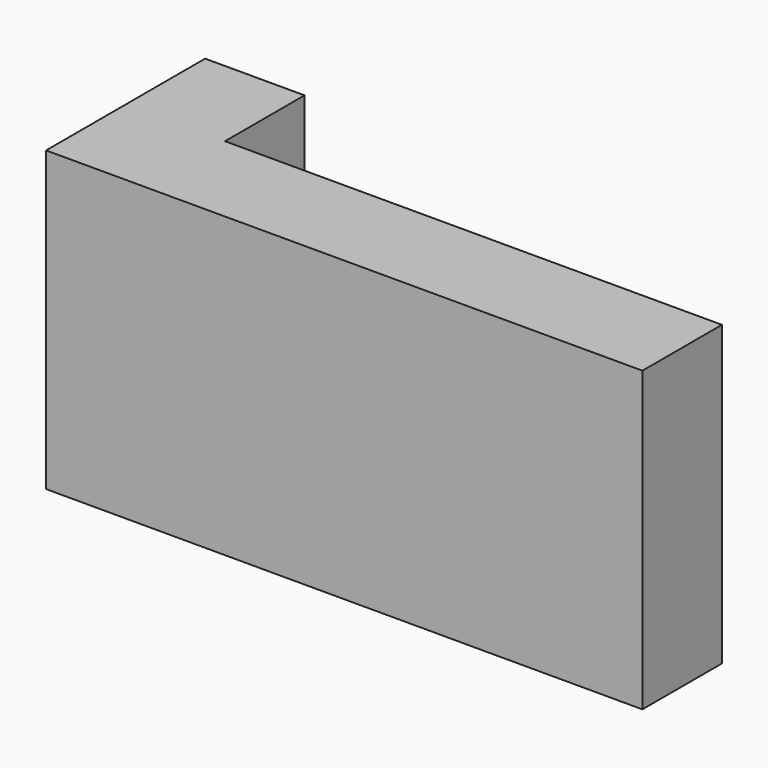
from build123d import *

# Parameters (mm, degrees)
F1_DEPTH = 50.8
F2_DEPTH = 25.4
F3_DEPTH = 25.4


with BuildPart() as f1:
    # F0 (on Top) → F1 (new body)
    with BuildSketch(Plane.XY):
        Polygon((-37.0331916732, 55.9852184538), (-62.4331916732, 55.9852184538), (-62.4331916732, 5.1852184538), (89.9668083268, 5.1852184538), (89.9668083268, 30.5852184538), (-37.0331916732, 30.5852184538), (-37.0331916732, 55.3826626255), align=None)
    extrude(amount=-F1_DEPTH)

    # F0 (on Top) → F3 (join)
    with BuildSketch(Plane.XY):
        Polygon((-37.0331916732, 55.9852184538), (-62.4331916732, 55.9852184538), (-62.4331916732, 5.1852184538), (89.9668083268, 5.1852184538), (89.9668083268, 30.5852184538), (-37.0331916732, 30.5852184538), (-37.0331916732, 55.3826626255), align=None)
    extrude(amount=F3_DEPTH)


with BuildPart() as f2:
    # F0 (on Top) → F2 (new body)
    with BuildSketch(Plane.XY):
        Polygon((89.9668083268, 30.5852184538), (-37.0331916732, 55.3826626255), (-37.0331916732, 30.5852184538), align=None)
    extrude(amount=-F2_DEPTH)


solid = Compound([f1.part, f2.part])
